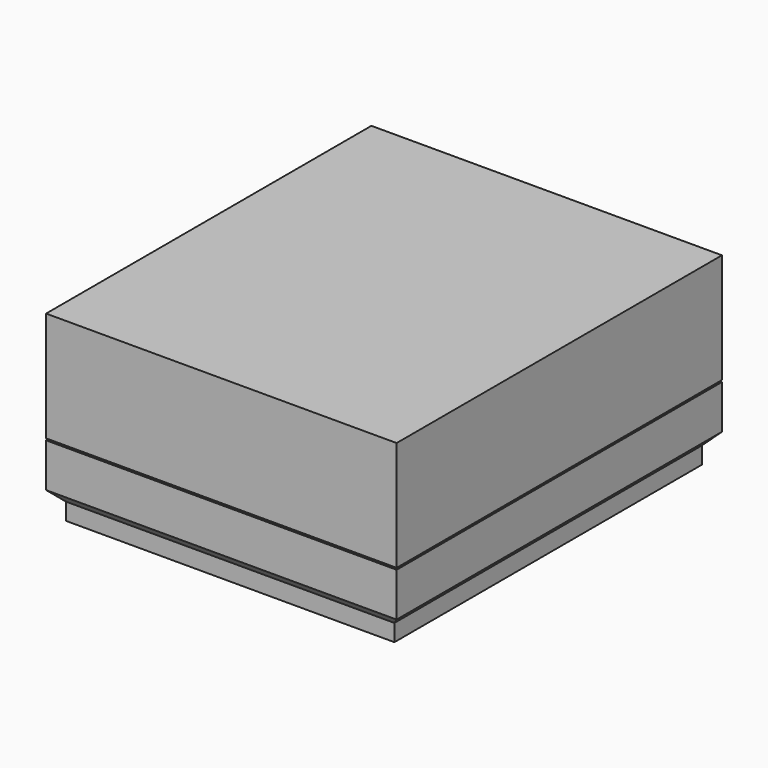
from build123d import *

# Parameters (mm, degrees)
F6_W          = 60
F6_H          = 69.6
F7_DEPTH      = 1
F8_W          = 60
F8_H          = 69.6
F8_W_2        = 53
F8_H_2        = 62.6
F9_DEPTH      = 14.6
F11_DEPTH     = 62.6
F14_W         = 60
F14_H         = 69.6
F14_W_2       = 56.2
F14_H_2       = 65.8
F15_DEPTH     = 3.3
F16_W         = 60
F16_H         = 69.6
F16_W_2       = 56.2
F16_H_2       = 65.8
F17_DEPTH     = 4.9
F18_T4_DEPTH  = 56.2
F18_T9_DEPTH  = 65.8
F18_T14_DEPTH = 56.2
F18_T19_DEPTH = 65.8
F18_T25_DEPTH = 61.3433659759
F18_T31_DEPTH = 70.9433659759
F18_T40_DEPTH = 61.3433659759
F18_T46_DEPTH = 70.9433659759
F18_T55_DEPTH = 61.3433659759
F18_T61_DEPTH = 70.9433659759
F18_T70_DEPTH = 70.9433659759
F18_T76_DEPTH = 61.3433659759
F19_W         = 60
F19_H         = 69.6
F19_W_2       = 56.8
F19_H_2       = 66.4
F20_DEPTH     = 3.2
F21_DEPTH     = 62.6


# Not quite as in the source:
# - a fillet or chamfer that OpenCascade refuses, or shapes differently, is made with other operations: its cross-section is extruded or revolved along the edge and cut away or added


with BuildPart() as f7:
    # F6 (on Top) → F7 (new body)
    with BuildSketch(Plane.XY):
        Rectangle(F6_W, F6_H)
    extrude(amount=F7_DEPTH)

    # F8 (on face) → F9 (join)
    with BuildSketch(Plane.XY.offset(1)):
        Rectangle(F8_W, F8_H)
        Rectangle(F8_W_2, F8_H_2, mode=Mode.SUBTRACT)
    extrude(amount=F9_DEPTH)

    # F10 (on face) → F11 (join, through all)
    with BuildSketch(Plane.XZ.offset(-31.3)):
        Polygon((2.8, 15.6), (0.8, 15.6), (0.8, 14.6), (0.8, 1), (2.8, 1), (2.8, 12.6), align=None)
    extrude(amount=F11_DEPTH)


with BuildPart() as f13_1:
    # F13: instance of F7
    add(f7.part.mirror(Plane(origin=(0.2291641245, 0, 15.7), x_dir=(1, 0, 0), z_dir=(0, 0, 1))))

    # F19 (on face) → F20 (join)
    with BuildSketch(Plane(origin=(0, 0, 15.8), x_dir=(1, 0, 0), z_dir=(0, 0, -1))):
        Rectangle(F19_W, F19_H)
        Rectangle(F19_W_2, F19_H_2, mode=Mode.SUBTRACT)
    extrude(amount=F20_DEPTH)


with BuildPart() as f7_1:
    add(f7.part)

    # F14 (on face) → F15 (cut)
    with BuildSketch(Plane.XY.offset(15.6)):
        Rectangle(F14_W, F14_H)
        Rectangle(F14_W_2, F14_H_2, mode=Mode.SUBTRACT)
    extrude(amount=-F15_DEPTH, mode=Mode.SUBTRACT)

    # F16 (on face) → F17 (cut)
    with BuildSketch(Plane(origin=(0, 0, 0), x_dir=(1, 0, 0), z_dir=(0, 0, -1))):
        Rectangle(F16_W, F16_H)
        Rectangle(F16_W_2, F16_H_2, mode=Mode.SUBTRACT)
    extrude(amount=-F17_DEPTH, mode=Mode.SUBTRACT)

    # F18: chamfer of 2 on 4 edges, made by hand


with BuildPart() as f18_tool2:
    # F18_s3 → F18_t4 (new body)
    with BuildSketch(Plane.YZ.offset(-28.1)):
        Polygon((-34.9, 4.9), (-32.9, 2.9), (-32.9, 4.9), align=None)
    extrude(amount=F18_T4_DEPTH)

    split(bisect_by=Plane.XZ.offset(34.8), keep=Keep.BOTTOM)


with BuildPart() as f7_2:
    add(f7_1.part)

    # F18_t1: union F18_tool2
    add(f18_tool2.part)


with BuildPart() as f18_tool7:
    # F18_s8 → F18_t9 (new body)
    with BuildSketch(Plane.XZ.offset(-32.9)):
        Polygon((-30.1, 4.9), (-28.1, 2.9), (-28.1, 4.9), align=None)
    extrude(amount=F18_T9_DEPTH)

    split(bisect_by=Plane.YZ.offset(-30), keep=Keep.TOP)


with BuildPart() as f7_3:
    add(f7_2.part)

    # F18_t6: union F18_tool7
    add(f18_tool7.part)


with BuildPart() as f18_tool12:
    # F18_s13 → F18_t14 (new body)
    with BuildSketch(Plane.YZ.offset(28.1)):
        Polygon((34.9, 4.9), (32.9, 2.9), (32.9, 4.9), align=None)
    extrude(amount=-F18_T14_DEPTH)

    split(bisect_by=Plane.XZ.offset(-34.8), keep=Keep.TOP)


with BuildPart() as f7_4:
    add(f7_3.part)

    # F18_t11: union F18_tool12
    add(f18_tool12.part)


with BuildPart() as f18_tool17:
    # F18_s18 → F18_t19 (new body)
    with BuildSketch(Plane.XZ.offset(32.9)):
        Polygon((30.1, 4.9), (28.1, 2.9), (28.1, 4.9), align=None)
    extrude(amount=-F18_T19_DEPTH)

    split(bisect_by=Plane.YZ.offset(30), keep=Keep.BOTTOM)


with BuildPart() as f7_5:
    add(f7_4.part)

    # F18_t16: union F18_tool17
    add(f18_tool17.part)


with BuildPart() as f18_tool23:
    # F18_s24 → F18_t25 (new body)
    with BuildSketch(Plane.YZ.offset(-33.2433659759)):
        Polygon((-34.9, 4.9), (-32.9, 2.9), (-32.9, 4.9), align=None)
    extrude(amount=F18_T25_DEPTH)

    split(bisect_by=Plane.XZ.offset(34.8), keep=Keep.BOTTOM)

    split(bisect_by=Plane.YZ.offset(-30), keep=Keep.TOP)

    split(bisect_by=Plane.YZ.offset(-28.1), keep=Keep.BOTTOM)


with BuildPart() as f18_tool29:
    # F18_s30 → F18_t31 (new body)
    with BuildSketch(Plane.XZ.offset(-32.9)):
        Polygon((-30.1, 4.9), (-28.1, 2.9), (-28.1, 4.9), align=None)
    extrude(amount=F18_T31_DEPTH)

    split(bisect_by=Plane.XZ.offset(34.8), keep=Keep.BOTTOM)

    split(bisect_by=Plane.YZ.offset(-30), keep=Keep.TOP)

    split(bisect_by=Plane.XZ.offset(32.9), keep=Keep.TOP)


with BuildPart() as f18_tool23_1:
    add(f18_tool23.part)

    # F18_t35: intersect F18_tool29
    add(f18_tool29.part, mode=Mode.INTERSECT)


with BuildPart() as f7_6:
    add(f7_5.part)

    # F18_t21: union F18_tool23
    add(f18_tool23_1.part)


with BuildPart() as f18_tool38:
    # F18_s39 → F18_t40 (new body)
    with BuildSketch(Plane.YZ.offset(-28.1)):
        Polygon((-34.9, 4.9), (-32.9, 2.9), (-32.9, 4.9), align=None)
    extrude(amount=F18_T40_DEPTH)

    split(bisect_by=Plane.XZ.offset(34.8), keep=Keep.BOTTOM)

    split(bisect_by=Plane.YZ.offset(30), keep=Keep.BOTTOM)

    split(bisect_by=Plane.YZ.offset(28.1), keep=Keep.TOP)


with BuildPart() as f18_tool44:
    # F18_s45 → F18_t46 (new body)
    with BuildSketch(Plane.XZ.offset(38.0433659759)):
        Polygon((30.1, 4.9), (28.1, 2.9), (28.1, 4.9), align=None)
    extrude(amount=-F18_T46_DEPTH)

    split(bisect_by=Plane.XZ.offset(34.8), keep=Keep.BOTTOM)

    split(bisect_by=Plane.YZ.offset(30), keep=Keep.BOTTOM)

    split(bisect_by=Plane.XZ.offset(32.9), keep=Keep.TOP)


with BuildPart() as f18_tool38_1:
    add(f18_tool38.part)

    # F18_t50: intersect F18_tool44
    add(f18_tool44.part, mode=Mode.INTERSECT)


with BuildPart() as f7_7:
    add(f7_6.part)

    # F18_t36: union F18_tool38
    add(f18_tool38_1.part)


with BuildPart() as f18_tool53:
    # F18_s54 → F18_t55 (new body)
    with BuildSketch(Plane.YZ.offset(28.1)):
        Polygon((34.9, 4.9), (32.9, 2.9), (32.9, 4.9), align=None)
    extrude(amount=-F18_T55_DEPTH)

    split(bisect_by=Plane.YZ.offset(-30), keep=Keep.TOP)

    split(bisect_by=Plane.XZ.offset(-34.8), keep=Keep.TOP)

    split(bisect_by=Plane.YZ.offset(-28.1), keep=Keep.BOTTOM)


with BuildPart() as f18_tool59:
    # F18_s60 → F18_t61 (new body)
    with BuildSketch(Plane.XZ.offset(-38.0433659759)):
        Polygon((-30.1, 4.9), (-28.1, 2.9), (-28.1, 4.9), align=None)
    extrude(amount=F18_T61_DEPTH)

    split(bisect_by=Plane.YZ.offset(-30), keep=Keep.TOP)

    split(bisect_by=Plane.XZ.offset(-34.8), keep=Keep.TOP)

    split(bisect_by=Plane.XZ.offset(-32.9), keep=Keep.BOTTOM)


with BuildPart() as f18_tool53_1:
    add(f18_tool53.part)

    # F18_t65: intersect F18_tool59
    add(f18_tool59.part, mode=Mode.INTERSECT)


with BuildPart() as f7_8:
    add(f7_7.part)

    # F18_t51: union F18_tool53
    add(f18_tool53_1.part)


with BuildPart() as f18_tool68:
    # F18_s69 → F18_t70 (new body)
    with BuildSketch(Plane.XZ.offset(32.9)):
        Polygon((30.1, 4.9), (28.1, 2.9), (28.1, 4.9), align=None)
    extrude(amount=-F18_T70_DEPTH)

    split(bisect_by=Plane.YZ.offset(30), keep=Keep.BOTTOM)

    split(bisect_by=Plane.XZ.offset(-34.8), keep=Keep.TOP)

    split(bisect_by=Plane.XZ.offset(-32.9), keep=Keep.BOTTOM)


with BuildPart() as f18_tool74:
    # F18_s75 → F18_t76 (new body)
    with BuildSketch(Plane.YZ.offset(33.2433659759)):
        Polygon((34.9, 4.9), (32.9, 2.9), (32.9, 4.9), align=None)
    extrude(amount=-F18_T76_DEPTH)

    split(bisect_by=Plane.YZ.offset(30), keep=Keep.BOTTOM)

    split(bisect_by=Plane.XZ.offset(-34.8), keep=Keep.TOP)

    split(bisect_by=Plane.YZ.offset(28.1), keep=Keep.TOP)


with BuildPart() as f18_tool68_1:
    add(f18_tool68.part)

    # F18_t80: intersect F18_tool74
    add(f18_tool74.part, mode=Mode.INTERSECT)


with BuildPart() as f7_9:
    add(f7_8.part)

    # F18_t66: union F18_tool68
    add(f18_tool68_1.part)

    # F10 (on face) → F21 (join, through all)
    with BuildSketch(Plane.XZ.offset(-31.3)):
        Polygon((14.4, 1), (2.8, 12.6), (2.8, 1), align=None)
        Polygon((26.5, 1), (26.5, 12.6), (14.9, 1), align=None)
        Polygon((-21.475, 1), (-25.6163476009, 14.6), (-26.5, 14.6), (-26.5, 1), align=None)
        Polygon((0.8, 1), (0.8, 14.6), (-0.0836523991, 14.6), (-4.225, 1), align=None)
    extrude(amount=F21_DEPTH)


solid = Compound([f13_1.part, f7_9.part])
